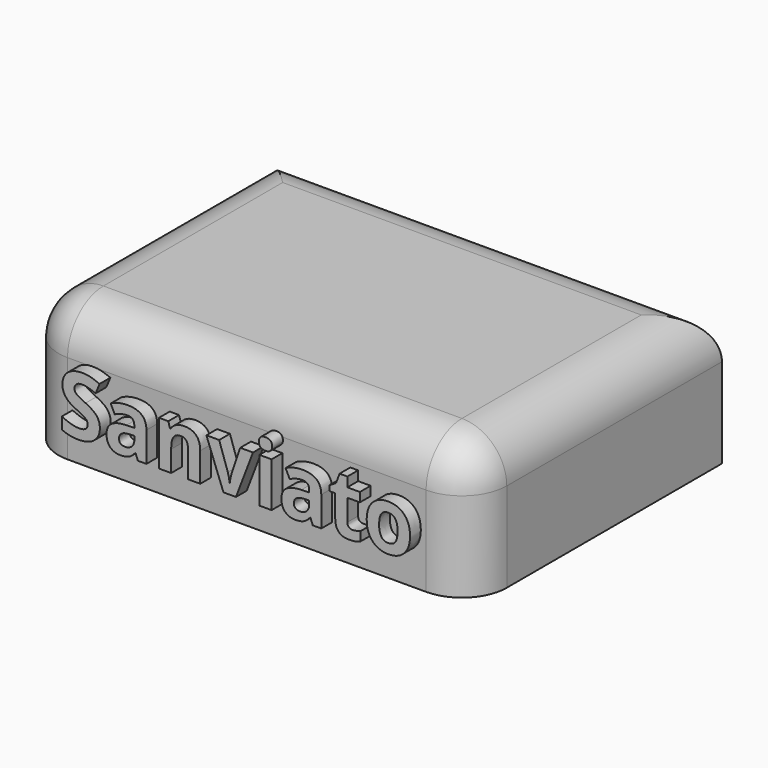
from build123d import *

# Parameters (mm, degrees)
F0_W         = 100
F0_H         = 70
F1_DEPTH     = 30
F2_R         = 10
F3_R         = 10
F4_TEXT_SIZE = 18.2736132052
F5_DEPTH     = 3


# Not quite as in the source:
# - Text() gives the source's letters only with a copy of the font that has no kerning and outlines rounded to 1/6400 em; it was checked with that copy


with BuildPart() as f1:
    # F0 (on Top) → F1 (new body)
    with BuildSketch(Plane.XY):
        with Locations((-0.7363804984, 11.0360253602)):
            Rectangle(F0_W, F0_H)
    extrude(amount=F1_DEPTH)

    # F2
    f2_edges = [f1.edges().sort_by_distance(p)[0] for p in [
        (-0.73638, -23.963975, 30),
    ]]
    fillet(f2_edges, radius=F2_R)

    # F3
    f3_edges = [f1.edges().sort_by_distance(p)[0] for p in [
        (49.26362, 16.036025, 30),
        (-50.73638, 16.036025, 30),
        (-0.73638, 46.036025, 30),
    ]]
    fillet(f3_edges, radius=F3_R)

    # F4 (on face) → F5 (join)
    with BuildSketch(Plane.XZ.offset(23.9639746398)):
        with Locations((-40.4692943662, 6.8429984923)):
            Text('Sanviato', F4_TEXT_SIZE, font='Open Sans', font_style=FontStyle.BOLD, text_align=(TextAlign.LEFT, TextAlign.BOTTOM))
    extrude(amount=F5_DEPTH)


solid = f1.part
